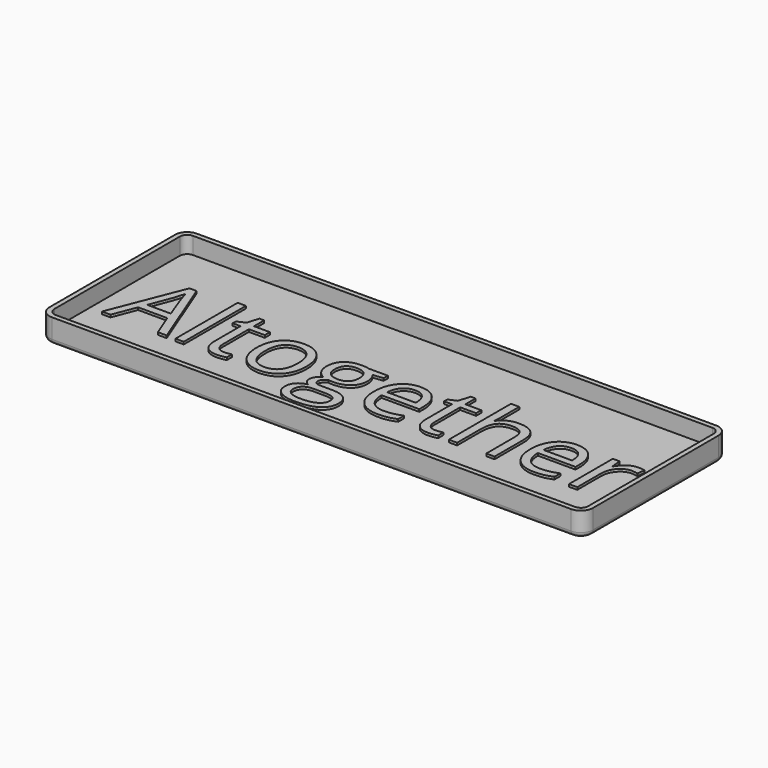
from build123d import *

# Parameters (mm, degrees)
F0_W         = 3.434615863
F0_H         = 32.1821521034
F1_DEPTH     = 3
F2_DEPTH     = 10
F0_TEXT_SIZE = 42.3536445532
F3_DEPTH     = 4
F4_R         = 2


# Not quite as in the source:
# - Text() gives the source's letters only with a copy of the font that has no kerning and outlines rounded to 1/6400 em; it was checked with that copy


with BuildPart() as f1:
    # F0 (on Top) → F1 (new body)
    with BuildSketch(Plane.XY):
        with BuildLine():
            ThreePointArc((-40.4605161873, 5), (-39.5818365309, 2.8786796564), (-37.4605161873, 2))
            Line((-37.4605161873, 2), (177.5394838127, 2))
            ThreePointArc((177.5394838127, 2), (179.6608041562, 2.8786796564), (180.5394838127, 5))
            Line((180.5394838127, 5), (180.5394838127, 70))
            ThreePointArc((180.5394838127, 70), (179.6608041562, 72.1213203436), (177.5394838127, 73))
            Line((177.5394838127, 73), (-37.4605161873, 73))
            ThreePointArc((-37.4605161873, 73), (-39.5818365309, 72.1213203436), (-40.4605161873, 70))
            Line((-40.4605161873, 70), (-40.4605161873, 5))
        make_face()
        Polygon((-7.739013755, 22.2526879609), (-11.3787800838, 22.2526879609), (-15.1442837949, 31.8682888258), (-27.2613967912, 31.8682888258), (-30.9805762036, 22.2526879609), (-34.5409294488, 22.2526879609), (-22.5892603765, 52.6149568999), (-19.6311230147, 52.6149568999), align=None, mode=Mode.SUBTRACT)
        with BuildLine():
            add(Edge.make_bspline(
                [(11.2671842382, 25.7700257859), (12.2399945115, 24.6747870087), (13.9341402937, 24.6747870087)],
                knots=[0, 0, 0, 1, 1, 1], degree=2))
            add(Edge.make_bspline(
                [(13.9341402937, 24.6747870087), (14.8473907543, 24.6747870087), (15.6944636454, 24.807142148)],
                knots=[0, 0, 0, 1, 1, 1], degree=2))
            add(Edge.make_bspline(
                [(15.6944636454, 24.807142148), (16.5415365365, 24.9394972872), (17.0378683086, 25.0850879404)],
                knots=[0, 0, 0, 1, 1, 1], degree=2))
            Line((17.0378683086, 25.0850879404), (17.0378683086, 22.4578384267))
            add(Edge.make_bspline(
                [(17.0378683086, 22.4578384267), (16.4819767238, 22.1931281482), (15.3966645821, 22.0144487103)],
                knots=[0, 0, 0, 1, 1, 1], degree=2))
            add(Edge.make_bspline(
                [(15.3966645821, 22.0144487103), (14.3113524405, 21.8357692723), (13.4378085216, 21.8357692723)],
                knots=[0, 0, 0, 1, 1, 1], degree=2))
            add(Edge.make_bspline(
                [(13.4378085216, 21.8357692723), (6.8663758589, 21.8357692723), (6.8663758589, 28.7645608109)],
                knots=[0, 0, 0, 1, 1, 1], degree=2))
            Line((6.8663758589, 28.7645608109), (6.8663758589, 42.2515494983))
            Line((6.8663758589, 42.2515494983), (3.6170571908, 42.2515494983))
            Line((3.6170571908, 42.2515494983), (3.6170571908, 43.9059887387))
            Line((3.6170571908, 43.9059887387), (6.8663758589, 45.3354242423))
            Line((6.8663758589, 45.3354242423), (8.3090468764, 50.1730045811))
            Line((8.3090468764, 50.1730045811), (10.2943739649, 50.1730045811))
            Line((10.2943739649, 50.1730045811), (10.2943739649, 44.9185055538))
            Line((10.2943739649, 44.9185055538), (16.8724243845, 44.9185055538))
            Line((16.8724243845, 44.9185055538), (16.8724243845, 42.2515494983))
            Line((16.8724243845, 42.2515494983), (10.2943739649, 42.2515494983))
            Line((10.2943739649, 42.2515494983), (10.2943739649, 28.9101514641))
            add(Edge.make_bspline(
                [(10.2943739649, 28.9101514641), (10.2943739649, 26.865264563), (11.2671842382, 25.7700257859)],
                knots=[0, 0, 0, 1, 1, 1], degree=2))
        make_face(mode=Mode.SUBTRACT)
        with BuildLine():
            add(Edge.make_bspline(
                [(38.323883575, 42.1688275363), (41.1265036482, 39.0022308302), (41.1265036482, 33.6087589067)],
                knots=[0, 0, 0, 1, 1, 1], degree=2))
            add(Edge.make_bspline(
                [(41.1265036482, 33.6087589067), (41.1265036482, 28.063078573), (38.3371190889, 24.9494239226)],
                knots=[0, 0, 0, 1, 1, 1], degree=2))
            add(Edge.make_bspline(
                [(38.3371190889, 24.9494239226), (35.5477345297, 21.8357692723), (30.6241233504, 21.8357692723)],
                knots=[0, 0, 0, 1, 1, 1], degree=2))
            add(Edge.make_bspline(
                [(30.6241233504, 21.8357692723), (27.5799551481, 21.8357692723), (25.2240336699, 23.265204776)],
                knots=[0, 0, 0, 1, 1, 1], degree=2))
            add(Edge.make_bspline(
                [(25.2240336699, 23.265204776), (22.8681121916, 24.6946402796), (21.5842673411, 27.3615963351)],
                knots=[0, 0, 0, 1, 1, 1], degree=2))
            add(Edge.make_bspline(
                [(21.5842673411, 27.3615963351), (20.3004224906, 30.0285523905), (20.3004224906, 33.6087589067)],
                knots=[0, 0, 0, 1, 1, 1], degree=2))
            add(Edge.make_bspline(
                [(20.3004224906, 33.6087589067), (20.3004224906, 39.1478214834), (23.0732626574, 42.2416228629)],
                knots=[0, 0, 0, 1, 1, 1], degree=2))
            add(Edge.make_bspline(
                [(23.0732626574, 42.2416228629), (25.8461028242, 45.3354242423), (30.7697140035, 45.3354242423)],
                knots=[0, 0, 0, 1, 1, 1], degree=2))
            add(Edge.make_bspline(
                [(30.7697140035, 45.3354242423), (35.5212635019, 45.3354242423), (38.323883575, 42.1688275363)],
                knots=[0, 0, 0, 1, 1, 1], degree=2))
        make_face(mode=Mode.SUBTRACT)
        with BuildLine():
            Line((57.8628110036, 44.9185055538), (65.698235246, 44.9185055538))
            Line((65.698235246, 44.9185055538), (65.698235246, 42.7478812704))
            Line((65.698235246, 42.7478812704), (61.5025773324, 42.2515494983))
            add(Edge.make_bspline(
                [(61.5025773324, 42.2515494983), (62.0783221881, 41.5302139895), (62.5349474184, 40.3588710073)],
                knots=[0, 0, 0, 1, 1, 1], degree=2))
            add(Edge.make_bspline(
                [(62.5349474184, 40.3588710073), (62.9915726488, 39.1875280252), (62.9915726488, 37.7250037367)],
                knots=[0, 0, 0, 1, 1, 1], degree=2))
            add(Edge.make_bspline(
                [(62.9915726488, 37.7250037367), (62.9915726488, 34.3896542281), (60.715064254, 32.4043271397)],
                knots=[0, 0, 0, 1, 1, 1], degree=2))
            add(Edge.make_bspline(
                [(60.715064254, 32.4043271397), (58.4385558593, 30.4190000513), (54.4679016824, 30.4190000513)],
                knots=[0, 0, 0, 1, 1, 1], degree=2))
            add(Edge.make_bspline(
                [(54.4679016824, 30.4190000513), (53.4553848673, 30.4190000513), (52.5686054345, 30.5844439753)],
                knots=[0, 0, 0, 1, 1, 1], degree=2))
            add(Edge.make_bspline(
                [(52.5686054345, 30.5844439753), (50.3781278803, 29.4263365071), (50.3781278803, 27.6726309123)],
                knots=[0, 0, 0, 1, 1, 1], degree=2))
            add(Edge.make_bspline(
                [(50.3781278803, 27.6726309123), (50.3781278803, 26.7395271807), (51.1424788093, 26.2961374643)],
                knots=[0, 0, 0, 1, 1, 1], degree=2))
            add(Edge.make_bspline(
                [(51.1424788093, 26.2961374643), (51.9068297384, 25.8527477479), (53.7664194445, 25.8527477479)],
                knots=[0, 0, 0, 1, 1, 1], degree=2))
            Line((53.7664194445, 25.8527477479), (57.7767801631, 25.8527477479))
            add(Edge.make_bspline(
                [(57.7767801631, 25.8527477479), (61.4628707907, 25.8527477479), (63.4349623652, 24.3008837404)],
                knots=[0, 0, 0, 1, 1, 1], degree=2))
            add(Edge.make_bspline(
                [(63.4349623652, 24.3008837404), (65.4070539397, 22.749019733), (65.4070539397, 19.7908823712)],
                knots=[0, 0, 0, 1, 1, 1], degree=2))
            add(Edge.make_bspline(
                [(65.4070539397, 19.7908823712), (65.4070539397, 16.0253786602), (62.3893567653, 14.0499782072)],
                knots=[0, 0, 0, 1, 1, 1], degree=2))
            add(Edge.make_bspline(
                [(62.3893567653, 14.0499782072), (59.3716595908, 12.0745777542), (53.5811222496, 12.0745777542)],
                knots=[0, 0, 0, 1, 1, 1], degree=2))
            add(Edge.make_bspline(
                [(53.5811222496, 12.0745777542), (49.1339895715, 12.0745777542), (46.7251260376, 13.7290169945)],
                knots=[0, 0, 0, 1, 1, 1], degree=2))
            add(Edge.make_bspline(
                [(46.7251260376, 13.7290169945), (44.3162625036, 15.3834562349), (44.3162625036, 18.4077711663)],
                knots=[0, 0, 0, 1, 1, 1], degree=2))
            add(Edge.make_bspline(
                [(44.3162625036, 18.4077711663), (44.3162625036, 20.4725113382), (45.6398138959, 21.9846688039)],
                knots=[0, 0, 0, 1, 1, 1], degree=2))
            add(Edge.make_bspline(
                [(45.6398138959, 21.9846688039), (46.9633652882, 23.4968262696), (49.3589933082, 24.0328645835)],
                knots=[0, 0, 0, 1, 1, 1], degree=2))
            add(Edge.make_bspline(
                [(49.3589933082, 24.0328645835), (48.4920671463, 24.4233122442), (47.9030867767, 25.2505318644)],
                knots=[0, 0, 0, 1, 1, 1], degree=2))
            add(Edge.make_bspline(
                [(47.9030867767, 25.2505318644), (47.3141064071, 26.0777514846), (47.3141064071, 27.1762991402)],
                knots=[0, 0, 0, 1, 1, 1], degree=2))
            add(Edge.make_bspline(
                [(47.3141064071, 27.1762991402), (47.3141064071, 28.413819692), (47.9758821033, 29.3469234235)],
                knots=[0, 0, 0, 1, 1, 1], degree=2))
            add(Edge.make_bspline(
                [(47.9758821033, 29.3469234235), (48.6376577994, 30.2800271551), (50.0670933031, 31.146953317)],
                knots=[0, 0, 0, 1, 1, 1], degree=2))
            add(Edge.make_bspline(
                [(50.0670933031, 31.146953317), (48.3067699513, 31.8682888258), (47.2016045388, 33.6054500282)],
                knots=[0, 0, 0, 1, 1, 1], degree=2))
            add(Edge.make_bspline(
                [(47.2016045388, 33.6054500282), (46.0964391262, 35.3426112306), (46.0964391262, 37.5794130835)],
                knots=[0, 0, 0, 1, 1, 1], degree=2))
            add(Edge.make_bspline(
                [(46.0964391262, 37.5794130835), (46.0964391262, 41.2985924959), (48.3299321007, 43.3170083691)],
                knots=[0, 0, 0, 1, 1, 1], degree=2))
            add(Edge.make_bspline(
                [(48.3299321007, 43.3170083691), (50.5634250752, 45.3354242423), (54.6531988773, 45.3354242423)],
                knots=[0, 0, 0, 1, 1, 1], degree=2))
            add(Edge.make_bspline(
                [(54.6531988773, 45.3354242423), (56.4333755, 45.3354242423), (57.8628110036, 44.9185055538)],
                knots=[0, 0, 0, 1, 1, 1], degree=2))
        make_face(mode=Mode.SUBTRACT)
        with BuildLine():
            add(Edge.make_bspline(
                [(83.8441248342, 22.1798926343), (82.2227743787, 21.8357692723), (79.9264127131, 21.8357692723)],
                knots=[0, 0, 0, 1, 1, 1], degree=2))
            add(Edge.make_bspline(
                [(79.9264127131, 21.8357692723), (74.9035351793, 21.8357692723), (71.9950309948, 24.8997907454)],
                knots=[0, 0, 0, 1, 1, 1], degree=2))
            add(Edge.make_bspline(
                [(71.9950309948, 24.8997907454), (69.0865268102, 27.9638122186), (69.0865268102, 33.3969906839)],
                knots=[0, 0, 0, 1, 1, 1], degree=2))
            add(Edge.make_bspline(
                [(69.0865268102, 33.3969906839), (69.0865268102, 38.8831112049), (71.7865716505, 42.1092677236)],
                knots=[0, 0, 0, 1, 1, 1], degree=2))
            add(Edge.make_bspline(
                [(71.7865716505, 42.1092677236), (74.4866164908, 45.3354242423), (79.0396332802, 45.3354242423)],
                knots=[0, 0, 0, 1, 1, 1], degree=2))
            add(Edge.make_bspline(
                [(79.0396332802, 45.3354242423), (83.2948510064, 45.3354242423), (85.776509867, 42.5328041692)],
                knots=[0, 0, 0, 1, 1, 1], degree=2))
            add(Edge.make_bspline(
                [(85.776509867, 42.5328041692), (88.2581687275, 39.730184096), (88.2581687275, 35.1374607648)],
                knots=[0, 0, 0, 1, 1, 1], degree=2))
            Line((88.2581687275, 35.1374607648), (88.2581687275, 32.9668364814))
            Line((88.2581687275, 32.9668364814), (72.6468800555, 32.9668364814))
            add(Edge.make_bspline(
                [(72.6468800555, 32.9668364814), (72.7527641669, 28.9763290337), (74.6652959287, 26.9082799832)],
                knots=[0, 0, 0, 1, 1, 1], degree=2))
            add(Edge.make_bspline(
                [(74.6652959287, 26.9082799832), (76.5778276906, 24.8402309328), (80.0521500953, 24.8402309328)],
                knots=[0, 0, 0, 1, 1, 1], degree=2))
            add(Edge.make_bspline(
                [(80.0521500953, 24.8402309328), (83.711769695, 24.8402309328), (87.2853584542, 26.3689327909)],
                knots=[0, 0, 0, 1, 1, 1], degree=2))
            Line((87.2853584542, 26.3689327909), (87.2853584542, 23.3049113177))
            add(Edge.make_bspline(
                [(87.2853584542, 23.3049113177), (85.4654752898, 22.5240159963), (83.8441248342, 22.1798926343)],
                knots=[0, 0, 0, 1, 1, 1], degree=2))
        make_face(mode=Mode.SUBTRACT)
        with BuildLine():
            add(Edge.make_bspline(
                [(98.7671667822, 25.7700257859), (99.7399770556, 24.6747870087), (101.4341228377, 24.6747870087)],
                knots=[0, 0, 0, 1, 1, 1], degree=2))
            add(Edge.make_bspline(
                [(101.4341228377, 24.6747870087), (102.3473732984, 24.6747870087), (103.1944461894, 24.807142148)],
                knots=[0, 0, 0, 1, 1, 1], degree=2))
            add(Edge.make_bspline(
                [(103.1944461894, 24.807142148), (104.0415190805, 24.9394972872), (104.5378508526, 25.0850879404)],
                knots=[0, 0, 0, 1, 1, 1], degree=2))
            Line((104.5378508526, 25.0850879404), (104.5378508526, 22.4578384267))
            add(Edge.make_bspline(
                [(104.5378508526, 22.4578384267), (103.9819592679, 22.1931281482), (102.8966471262, 22.0144487103)],
                knots=[0, 0, 0, 1, 1, 1], degree=2))
            add(Edge.make_bspline(
                [(102.8966471262, 22.0144487103), (101.8113349845, 21.8357692723), (100.9377910656, 21.8357692723)],
                knots=[0, 0, 0, 1, 1, 1], degree=2))
            add(Edge.make_bspline(
                [(100.9377910656, 21.8357692723), (94.3663584029, 21.8357692723), (94.3663584029, 28.7645608109)],
                knots=[0, 0, 0, 1, 1, 1], degree=2))
            Line((94.3663584029, 28.7645608109), (94.3663584029, 42.2515494983))
            Line((94.3663584029, 42.2515494983), (91.1170397348, 42.2515494983))
            Line((91.1170397348, 42.2515494983), (91.1170397348, 43.9059887387))
            Line((91.1170397348, 43.9059887387), (94.3663584029, 45.3354242423))
            Line((94.3663584029, 45.3354242423), (95.8090294205, 50.1730045811))
            Line((95.8090294205, 50.1730045811), (97.7943565089, 50.1730045811))
            Line((97.7943565089, 50.1730045811), (97.7943565089, 44.9185055538))
            Line((97.7943565089, 44.9185055538), (104.3724069286, 44.9185055538))
            Line((104.3724069286, 44.9185055538), (104.3724069286, 42.2515494983))
            Line((104.3724069286, 42.2515494983), (97.7943565089, 42.2515494983))
            Line((97.7943565089, 42.2515494983), (97.7943565089, 28.9101514641))
            add(Edge.make_bspline(
                [(97.7943565089, 28.9101514641), (97.7943565089, 26.865264563), (98.7671667822, 25.7700257859)],
                knots=[0, 0, 0, 1, 1, 1], degree=2))
        make_face(mode=Mode.SUBTRACT)
        with BuildLine():
            add(Edge.make_bspline(
                [(148.5525524031, 22.1798926343), (146.9312019475, 21.8357692723), (144.6348402819, 21.8357692723)],
                knots=[0, 0, 0, 1, 1, 1], degree=2))
            add(Edge.make_bspline(
                [(144.6348402819, 21.8357692723), (139.6119627482, 21.8357692723), (136.7034585637, 24.8997907454)],
                knots=[0, 0, 0, 1, 1, 1], degree=2))
            add(Edge.make_bspline(
                [(136.7034585637, 24.8997907454), (133.7949543791, 27.9638122186), (133.7949543791, 33.3969906839)],
                knots=[0, 0, 0, 1, 1, 1], degree=2))
            add(Edge.make_bspline(
                [(133.7949543791, 33.3969906839), (133.7949543791, 38.8831112049), (136.4949992194, 42.1092677236)],
                knots=[0, 0, 0, 1, 1, 1], degree=2))
            add(Edge.make_bspline(
                [(136.4949992194, 42.1092677236), (139.1950440596, 45.3354242423), (143.7480608491, 45.3354242423)],
                knots=[0, 0, 0, 1, 1, 1], degree=2))
            add(Edge.make_bspline(
                [(143.7480608491, 45.3354242423), (148.0032785753, 45.3354242423), (150.4849374358, 42.5328041692)],
                knots=[0, 0, 0, 1, 1, 1], degree=2))
            add(Edge.make_bspline(
                [(150.4849374358, 42.5328041692), (152.9665962964, 39.730184096), (152.9665962964, 35.1374607648)],
                knots=[0, 0, 0, 1, 1, 1], degree=2))
            Line((152.9665962964, 35.1374607648), (152.9665962964, 32.9668364814))
            Line((152.9665962964, 32.9668364814), (137.3553076244, 32.9668364814))
            add(Edge.make_bspline(
                [(137.3553076244, 32.9668364814), (137.4611917357, 28.9763290337), (139.3737234976, 26.9082799832)],
                knots=[0, 0, 0, 1, 1, 1], degree=2))
            add(Edge.make_bspline(
                [(139.3737234976, 26.9082799832), (141.2862552594, 24.8402309328), (144.7605776642, 24.8402309328)],
                knots=[0, 0, 0, 1, 1, 1], degree=2))
            add(Edge.make_bspline(
                [(144.7605776642, 24.8402309328), (148.4201972639, 24.8402309328), (151.993786023, 26.3689327909)],
                knots=[0, 0, 0, 1, 1, 1], degree=2))
            Line((151.993786023, 26.3689327909), (151.993786023, 23.3049113177))
            add(Edge.make_bspline(
                [(151.993786023, 23.3049113177), (150.1739028586, 22.5240159963), (148.5525524031, 22.1798926343)],
                knots=[0, 0, 0, 1, 1, 1], degree=2))
        make_face(mode=Mode.SUBTRACT)
        with BuildLine():
            add(Edge.make_bspline(
                [(165.2557709737, 44.1343013538), (167.0359475964, 45.3354242423), (169.166865338, 45.3354242423)],
                knots=[0, 0, 0, 1, 1, 1], degree=2))
            add(Edge.make_bspline(
                [(169.166865338, 45.3354242423), (170.6757139252, 45.3354242423), (171.8735279352, 45.0839494778)],
                knots=[0, 0, 0, 1, 1, 1], degree=2))
            Line((171.8735279352, 45.0839494778), (171.397049434, 41.9008083794))
            add(Edge.make_bspline(
                [(171.397049434, 41.9008083794), (169.9940849581, 42.2118429565), (168.9153905734, 42.2118429565)],
                knots=[0, 0, 0, 1, 1, 1], degree=2))
            add(Edge.make_bspline(
                [(168.9153905734, 42.2118429565), (166.1624036775, 42.2118429565), (164.2101653738, 39.9783499821)],
                knots=[0, 0, 0, 1, 1, 1], degree=2))
            add(Edge.make_bspline(
                [(164.2101653738, 39.9783499821), (162.2579270702, 37.7448570076), (162.2579270702, 34.416125256)],
                knots=[0, 0, 0, 1, 1, 1], degree=2))
            Line((162.2579270702, 34.416125256), (162.2579270702, 22.2526879609))
            Line((162.2579270702, 22.2526879609), (158.8233112072, 22.2526879609))
            Line((158.8233112072, 22.2526879609), (158.8233112072, 44.9185055538))
            Line((158.8233112072, 44.9185055538), (161.6557111867, 44.9185055538))
            Line((161.6557111867, 44.9185055538), (162.0527766044, 40.7228476402))
            Line((162.0527766044, 40.7228476402), (162.2182205284, 40.7228476402))
            add(Edge.make_bspline(
                [(162.2182205284, 40.7228476402), (163.4755943511, 42.9331784653), (165.2557709737, 44.1343013538)],
                knots=[0, 0, 0, 1, 1, 1], degree=2))
        make_face(mode=Mode.SUBTRACT)
        with Locations((-2.3819394947, 38.3437640126)):
            Rectangle(F0_W, F0_H, mode=Mode.SUBTRACT)
        with BuildLine():
            Line((128.0110347948, 22.2526879609), (124.5764189318, 22.2526879609))
            Line((124.5764189318, 22.2526879609), (124.5764189318, 36.9176373874))
            add(Edge.make_bspline(
                [(124.5764189318, 36.9176373874), (124.5764189318, 39.6838597973), (123.3157362307, 41.0504266098)],
                knots=[0, 0, 0, 1, 1, 1], degree=2))
            add(Edge.make_bspline(
                [(123.3157362307, 41.0504266098), (122.0550535295, 42.4169934223), (119.3616264462, 42.4169934223)],
                knots=[0, 0, 0, 1, 1, 1], degree=2))
            add(Edge.make_bspline(
                [(119.3616264462, 42.4169934223), (115.788037687, 42.4169934223), (114.1435250821, 40.4713728757)],
                knots=[0, 0, 0, 1, 1, 1], degree=2))
            add(Edge.make_bspline(
                [(114.1435250821, 40.4713728757), (112.4990124772, 38.525752329), (112.4990124772, 34.1050906788)],
                knots=[0, 0, 0, 1, 1, 1], degree=2))
            Line((112.4990124772, 34.1050906788), (112.4990124772, 22.2526879609))
            Line((112.4990124772, 22.2526879609), (109.0643966142, 22.2526879609))
            Line((109.0643966142, 22.2526879609), (109.0643966142, 54.4348400643))
            Line((109.0643966142, 54.4348400643), (112.4990124772, 54.4348400643))
            Line((112.4990124772, 54.4348400643), (112.4990124772, 44.6935018171))
            add(Edge.make_bspline(
                [(112.4990124772, 44.6935018171), (112.4990124772, 42.9331784653), (112.3335685532, 41.7750709971)],
                knots=[0, 0, 0, 1, 1, 1], degree=2))
            Line((112.3335685532, 41.7750709971), (112.538719019, 41.7750709971))
            add(Edge.make_bspline(
                [(112.538719019, 41.7750709971), (113.5512358341, 43.4096569666), (115.4240610542, 44.3493784551)],
                knots=[0, 0, 0, 1, 1, 1], degree=2))
            add(Edge.make_bspline(
                [(115.4240610542, 44.3493784551), (117.2968862743, 45.2890999436), (119.6925142943, 45.2890999436)],
                knots=[0, 0, 0, 1, 1, 1], degree=2))
            add(Edge.make_bspline(
                [(119.6925142943, 45.2890999436), (123.8484656661, 45.2890999436), (125.9297502304, 43.3136994906)],
                knots=[0, 0, 0, 1, 1, 1], degree=2))
            add(Edge.make_bspline(
                [(125.9297502304, 43.3136994906), (128.0110347948, 41.3382990376), (128.0110347948, 37.0367570127)],
                knots=[0, 0, 0, 1, 1, 1], degree=2))
            Line((128.0110347948, 37.0367570127), (128.0110347948, 22.2526879609))
        make_face(mode=Mode.SUBTRACT)
    extrude(amount=F1_DEPTH)

    # F0 (on Top) → F2 (join)
    with BuildSketch(Plane.XY):
        with BuildLine():
            Line((177.5394838127, 75), (-37.4605161873, 75))
            ThreePointArc((-37.4605161873, 75), (-40.9960500933, 73.5355339059), (-42.4605161873, 70))
            Line((-42.4605161873, 70), (-42.4605161873, 5))
            ThreePointArc((-42.4605161873, 5), (-40.9960500933, 1.4644660941), (-37.4605161873, 0))
            Line((-37.4605161873, 0), (177.5394838127, 0))
            ThreePointArc((177.5394838127, 0), (181.0750177186, 1.4644660941), (182.5394838127, 5))
            Line((182.5394838127, 5), (182.5394838127, 70))
            ThreePointArc((182.5394838127, 70), (181.0750177186, 73.5355339059), (177.5394838127, 75))
        make_face()
        with BuildLine():
            Line((177.5394838127, 2), (-37.4605161873, 2))
            ThreePointArc((-37.4605161873, 2), (-39.5818365309, 2.8786796564), (-40.4605161873, 5))
            Line((-40.4605161873, 5), (-40.4605161873, 70))
            ThreePointArc((-40.4605161873, 70), (-39.5818365309, 72.1213203436), (-37.4605161873, 73))
            Line((-37.4605161873, 73), (177.5394838127, 73))
            ThreePointArc((177.5394838127, 73), (179.6608041562, 72.1213203436), (180.5394838127, 70))
            Line((180.5394838127, 70), (180.5394838127, 5))
            ThreePointArc((180.5394838127, 5), (179.6608041562, 2.8786796564), (177.5394838127, 2))
        make_face(mode=Mode.SUBTRACT)
    extrude(amount=F2_DEPTH)



with BuildPart() as f1b:
    # F0 (on Top) → F1, piece 2 (new body)
    with BuildSketch(Plane.XY):
        with BuildLine():
            Line((-26.0172584825, 35.0315766534), (-16.2362136935, 35.0315766534))
            Line((-16.2362136935, 35.0315766534), (-19.756860397, 44.4023205108))
            add(Edge.make_bspline(
                [(-19.756860397, 44.4023205108), (-20.438489364, 46.1824971334), (-21.1598248728, 48.7634223484)],
                knots=[0, 0, 0, 1, 1, 1], degree=2))
            add(Edge.make_bspline(
                [(-21.1598248728, 48.7634223484), (-21.6164501031, 46.7780952599), (-22.4635229942, 44.4023205108)],
                knots=[0, 0, 0, 1, 1, 1], degree=2))
            Line((-22.4635229942, 44.4023205108), (-26.0172584825, 35.0315766534))
        make_face()
    extrude(amount=F1_DEPTH)


with BuildPart() as f1c:
    # F0 (on Top) → F1, piece 3 (new body)
    with BuildSketch(Plane.XY):
        with BuildLine():
            add(Edge.make_bspline(
                [(25.5780836673, 40.2033537187), (23.8607757358, 37.9897140151), (23.8607757358, 33.6087589067)],
                knots=[0, 0, 0, 1, 1, 1], degree=2))
            add(Edge.make_bspline(
                [(23.8607757358, 33.6087589067), (23.8607757358, 29.260892583), (25.5979369382, 26.9876930668)],
                knots=[0, 0, 0, 1, 1, 1], degree=2))
            add(Edge.make_bspline(
                [(25.5979369382, 26.9876930668), (27.3350981406, 24.7144935505), (30.7035364339, 24.7144935505)],
                knots=[0, 0, 0, 1, 1, 1], degree=2))
            add(Edge.make_bspline(
                [(30.7035364339, 24.7144935505), (34.0785924843, 24.7144935505), (35.8256803221, 26.9777664313)],
                knots=[0, 0, 0, 1, 1, 1], degree=2))
            add(Edge.make_bspline(
                [(35.8256803221, 26.9777664313), (37.5727681599, 29.2410393121), (37.5727681599, 33.6087589067)],
                knots=[0, 0, 0, 1, 1, 1], degree=2))
            add(Edge.make_bspline(
                [(37.5727681599, 33.6087589067), (37.5727681599, 37.9301542025), (35.8256803221, 40.1735738124)],
                knots=[0, 0, 0, 1, 1, 1], degree=2))
            add(Edge.make_bspline(
                [(35.8256803221, 40.1735738124), (34.0785924843, 42.4169934223), (30.6638298922, 42.4169934223)],
                knots=[0, 0, 0, 1, 1, 1], degree=2))
            add(Edge.make_bspline(
                [(30.6638298922, 42.4169934223), (27.2953915988, 42.4169934223), (25.5780836673, 40.2033537187)],
                knots=[0, 0, 0, 1, 1, 1], degree=2))
        make_face()
    extrude(amount=F1_DEPTH)


with BuildPart() as f1d:
    # F0 (on Top) → F1, piece 4 (new body)
    with BuildSketch(Plane.XY):
        with BuildLine():
            add(Edge.make_bspline(
                [(48.9288391057, 21.6537809559), (47.6251409843, 20.5386889079), (47.6251409843, 18.447477708)],
                knots=[0, 0, 0, 1, 1, 1], degree=2))
            add(Edge.make_bspline(
                [(47.6251409843, 18.447477708), (47.6251409843, 16.6077412728), (49.1770049918, 15.6547842703)],
                knots=[0, 0, 0, 1, 1, 1], degree=2))
            add(Edge.make_bspline(
                [(49.1770049918, 15.6547842703), (50.7288689992, 14.7018272679), (53.6208287914, 14.7018272679)],
                knots=[0, 0, 0, 1, 1, 1], degree=2))
            add(Edge.make_bspline(
                [(53.6208287914, 14.7018272679), (57.9422240872, 14.7018272679), (60.0201997731, 15.9955987538)],
                knots=[0, 0, 0, 1, 1, 1], degree=2))
            add(Edge.make_bspline(
                [(60.0201997731, 15.9955987538), (62.098175459, 17.2893702398), (62.098175459, 19.4997010649)],
                knots=[0, 0, 0, 1, 1, 1], degree=2))
            add(Edge.make_bspline(
                [(62.098175459, 19.4997010649), (62.098175459, 21.3394375002), (60.9632301401, 22.054155252)],
                knots=[0, 0, 0, 1, 1, 1], degree=2))
            add(Edge.make_bspline(
                [(60.9632301401, 22.054155252), (59.8282848212, 22.7688730039), (56.6848502645, 22.7688730039)],
                knots=[0, 0, 0, 1, 1, 1], degree=2))
            Line((56.6848502645, 22.7688730039), (52.5686054345, 22.7688730039))
            add(Edge.make_bspline(
                [(52.5686054345, 22.7688730039), (50.2325372271, 22.7688730039), (48.9288391057, 21.6537809559)],
                knots=[0, 0, 0, 1, 1, 1], degree=2))
        make_face()
    extrude(amount=F1_DEPTH)


with BuildPart() as f1e:
    # F0 (on Top) → F1, piece 5 (new body)
    with BuildSketch(Plane.XY):
        with BuildLine():
            add(Edge.make_bspline(
                [(50.7884288119, 41.526905111), (49.4847306905, 40.2265158681), (49.4847306905, 37.6588261671)],
                knots=[0, 0, 0, 1, 1, 1], degree=2))
            add(Edge.make_bspline(
                [(49.4847306905, 37.6588261671), (49.4847306905, 35.2830514179), (50.8281353536, 34.0620752585)],
                knots=[0, 0, 0, 1, 1, 1], degree=2))
            add(Edge.make_bspline(
                [(50.8281353536, 34.0620752585), (52.1715400168, 32.8410990992), (54.5737857938, 32.8410990992)],
                knots=[0, 0, 0, 1, 1, 1], degree=2))
            add(Edge.make_bspline(
                [(54.5737857938, 32.8410990992), (59.5966633275, 32.8410990992), (59.5966633275, 37.7250037367)],
                knots=[0, 0, 0, 1, 1, 1], degree=2))
            add(Edge.make_bspline(
                [(59.5966633275, 37.7250037367), (59.5966633275, 42.827294354), (54.5142259812, 42.827294354)],
                knots=[0, 0, 0, 1, 1, 1], degree=2))
            add(Edge.make_bspline(
                [(54.5142259812, 42.827294354), (52.0921269333, 42.827294354), (50.7884288119, 41.526905111)],
                knots=[0, 0, 0, 1, 1, 1], degree=2))
        make_face()
    extrude(amount=F1_DEPTH)


with BuildPart() as f1f:
    # F0 (on Top) → F1, piece 6 (new body)
    with BuildSketch(Plane.XY):
        with BuildLine():
            add(Edge.make_bspline(
                [(83.1327159609, 40.7294653972), (81.6867360648, 42.4566999641), (78.9933089815, 42.4566999641)],
                knots=[0, 0, 0, 1, 1, 1], degree=2))
            add(Edge.make_bspline(
                [(78.9933089815, 42.4566999641), (76.2667931134, 42.4566999641), (74.6421337794, 40.67983222)],
                knots=[0, 0, 0, 1, 1, 1], degree=2))
            add(Edge.make_bspline(
                [(74.6421337794, 40.67983222), (73.0174744453, 38.9029644758), (72.726293139, 35.7595299191)],
                knots=[0, 0, 0, 1, 1, 1], degree=2))
            Line((72.726293139, 35.7595299191), (84.5786958569, 35.7595299191))
            add(Edge.make_bspline(
                [(84.5786958569, 35.7595299191), (84.5786958569, 39.0022308302), (83.1327159609, 40.7294653972)],
                knots=[0, 0, 0, 1, 1, 1], degree=2))
        make_face()
    extrude(amount=F1_DEPTH)


with BuildPart() as f1g:
    # F0 (on Top) → F1, piece 7 (new body)
    with BuildSketch(Plane.XY):
        with BuildLine():
            add(Edge.make_bspline(
                [(147.8411435297, 40.7294653972), (146.3951636337, 42.4566999641), (143.7017365504, 42.4566999641)],
                knots=[0, 0, 0, 1, 1, 1], degree=2))
            add(Edge.make_bspline(
                [(143.7017365504, 42.4566999641), (140.9752206823, 42.4566999641), (139.3505613482, 40.67983222)],
                knots=[0, 0, 0, 1, 1, 1], degree=2))
            add(Edge.make_bspline(
                [(139.3505613482, 40.67983222), (137.7259020142, 38.9029644758), (137.4347207079, 35.7595299191)],
                knots=[0, 0, 0, 1, 1, 1], degree=2))
            Line((137.4347207079, 35.7595299191), (149.2871234258, 35.7595299191))
            add(Edge.make_bspline(
                [(149.2871234258, 35.7595299191), (149.2871234258, 39.0022308302), (147.8411435297, 40.7294653972)],
                knots=[0, 0, 0, 1, 1, 1], degree=2))
        make_face()
    extrude(amount=F1_DEPTH)


with BuildPart() as f1_1:
    add(f1.part)

    add(f1b.part)  # F3 merges F1b

    add(f1c.part)  # F3 merges F1c

    add(f1d.part)  # F3 merges F1d

    add(f1e.part)  # F3 merges F1e

    add(f1f.part)  # F3 merges F1f

    add(f1g.part)  # F3 merges F1g
    # F0 (on Top) → F3 (join)
    with BuildSketch(Plane.XY):
        with Locations((-34.5409294488, 22.2526879609)):
            Text('Altogether', F0_TEXT_SIZE, font='Open Sans', text_align=(TextAlign.LEFT, TextAlign.BOTTOM))
    extrude(amount=F3_DEPTH)

    # F4
    f4_edges = [f1_1.edges().sort_by_distance(p)[0] for p in [
        (70.039484, 75, 0),
    ]]
    fillet(f4_edges, radius=F4_R)


solid = f1_1.part
